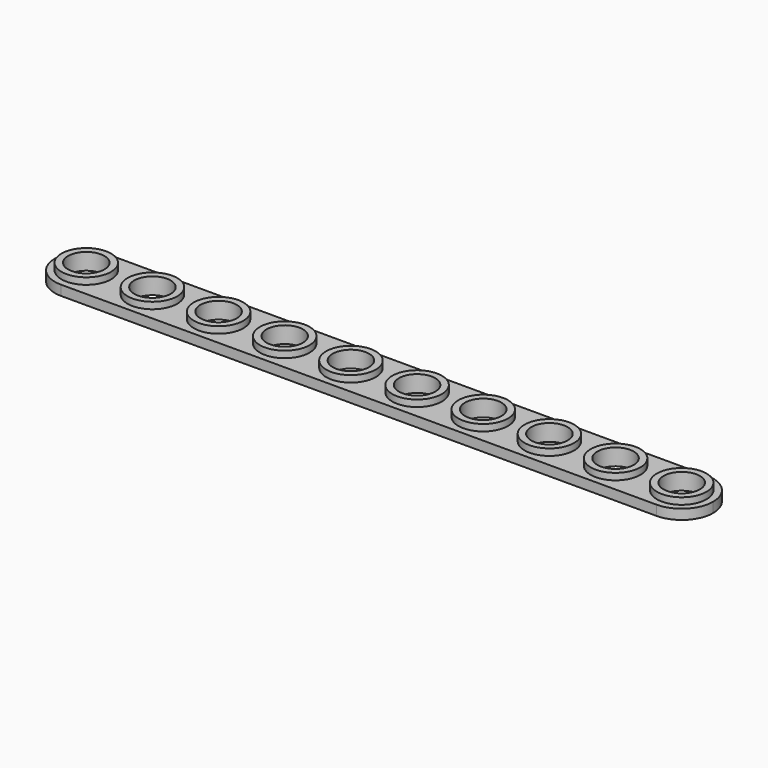
from build123d import *

# Parameters (mm, degrees)
F2_R     = 7.5
F2_R_2   = 5.5
F3_DEPTH = 3
F4_DEPTH = 5


# Not quite as in the source:
# - a feature names something its author has since deleted; it is built from what else it names


with BuildPart() as f3:
    # F2 (on Top) → F3 (new body)
    with BuildSketch(Plane.XY):
        with BuildLine():
            Line((180, 9.5), (0, 9.5))
            ThreePointArc((0, 9.5), (-6.7175144213, 6.7175144213), (-9.5, 0))
            ThreePointArc((-9.5, 0), (-6.7175144213, -6.7175144213), (0, -9.5))
            Line((0, -9.5), (180, -9.5))
            ThreePointArc((180, -9.5), (186.7175144213, -6.7175144213), (189.5, 0))
            ThreePointArc((189.5, 0), (186.7175144213, 6.7175144213), (180, 9.5))
        make_face()
        Circle(F2_R, mode=Mode.SUBTRACT)
        with Locations((20, 0)):
            Circle(F2_R, mode=Mode.SUBTRACT)
        with Locations((40, 0)):
            Circle(F2_R, mode=Mode.SUBTRACT)
        with Locations((60, 0)):
            Circle(F2_R, mode=Mode.SUBTRACT)
        with Locations((80, 0)):
            Circle(F2_R, mode=Mode.SUBTRACT)
        with Locations((100, 0)):
            Circle(F2_R, mode=Mode.SUBTRACT)
        with Locations((120, 0)):
            Circle(F2_R, mode=Mode.SUBTRACT)
        with Locations((140, 0)):
            Circle(F2_R, mode=Mode.SUBTRACT)
        with Locations((160, 0)):
            Circle(F2_R, mode=Mode.SUBTRACT)
        with Locations((180, 0)):
            Circle(F2_R, mode=Mode.SUBTRACT)
        Circle(F2_R)
        Circle(F2_R_2, mode=Mode.SUBTRACT)
        with Locations((20, 0)):
            Circle(F2_R)
        with Locations((20, 0)):
            Circle(F2_R_2, mode=Mode.SUBTRACT)
        with Locations((40, 0)):
            Circle(F2_R)
        with Locations((40, 0)):
            Circle(F2_R_2, mode=Mode.SUBTRACT)
        with Locations((60, 0)):
            Circle(F2_R)
        with Locations((60, 0)):
            Circle(F2_R_2, mode=Mode.SUBTRACT)
        with Locations((80, 0)):
            Circle(F2_R)
        with Locations((80, 0)):
            Circle(F2_R_2, mode=Mode.SUBTRACT)
        with Locations((100, 0)):
            Circle(F2_R)
        with Locations((100, 0)):
            Circle(F2_R_2, mode=Mode.SUBTRACT)
        with Locations((120, 0)):
            Circle(F2_R)
        with Locations((120, 0)):
            Circle(F2_R_2, mode=Mode.SUBTRACT)
        with Locations((140, 0)):
            Circle(F2_R)
        with Locations((140, 0)):
            Circle(F2_R_2, mode=Mode.SUBTRACT)
        with Locations((160, 0)):
            Circle(F2_R)
        with Locations((160, 0)):
            Circle(F2_R_2, mode=Mode.SUBTRACT)
        with Locations((180, 0)):
            Circle(F2_R)
        with Locations((180, 0)):
            Circle(F2_R_2, mode=Mode.SUBTRACT)
    extrude(amount=F3_DEPTH)

    # F2 (on Top) → F4 (join)
    with BuildSketch(Plane.XY):
        Circle(F2_R)
        Circle(F2_R_2, mode=Mode.SUBTRACT)
        with Locations((20, 0)):
            Circle(F2_R)
        with Locations((20, 0)):
            Circle(F2_R_2, mode=Mode.SUBTRACT)
        with Locations((40, 0)):
            Circle(F2_R)
        with Locations((40, 0)):
            Circle(F2_R_2, mode=Mode.SUBTRACT)
        with Locations((60, 0)):
            Circle(F2_R)
        with Locations((60, 0)):
            Circle(F2_R_2, mode=Mode.SUBTRACT)
        with Locations((80, 0)):
            Circle(F2_R)
        with Locations((80, 0)):
            Circle(F2_R_2, mode=Mode.SUBTRACT)
        with Locations((100, 0)):
            Circle(F2_R)
        with Locations((100, 0)):
            Circle(F2_R_2, mode=Mode.SUBTRACT)
        with Locations((120, 0)):
            Circle(F2_R)
        with Locations((120, 0)):
            Circle(F2_R_2, mode=Mode.SUBTRACT)
        with Locations((140, 0)):
            Circle(F2_R)
        with Locations((140, 0)):
            Circle(F2_R_2, mode=Mode.SUBTRACT)
        with Locations((160, 0)):
            Circle(F2_R)
        with Locations((160, 0)):
            Circle(F2_R_2, mode=Mode.SUBTRACT)
        with Locations((180, 0)):
            Circle(F2_R)
        with Locations((180, 0)):
            Circle(F2_R_2, mode=Mode.SUBTRACT)
    extrude(amount=F4_DEPTH)


solid = f3.part
